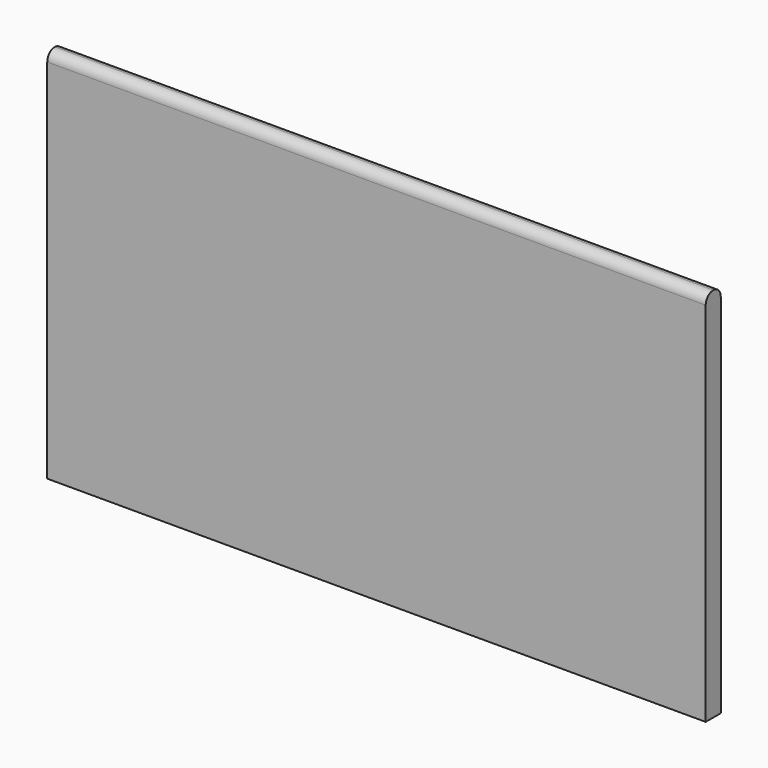
from build123d import *

# Parameters (mm, degrees)
F0_W     = 92.5
F0_H     = 20
F1_DEPTH = 1.4
F2_W     = 2
F2_H     = 2
F3_DEPTH = 25
F4_R     = 0.8
F6_W     = 70
F6_H     = 40
F7_DEPTH = 2
F8_R     = 0.99999


# Not quite as in the source:
# - a fillet or chamfer is up to 0.001 mm smaller than in the source, because OpenCascade refuses the exact size


with BuildPart() as f1:
    # F0 (on Top) → F1 (new body)
    with BuildSketch(Plane.XY):
        with Locations((46.25, 10)):
            Rectangle(F0_W, F0_H)
    extrude(amount=F1_DEPTH)

    # F2 (on face) → F3 (cut)
    with BuildSketch(Plane.XY.offset(1.4)):
        with Locations((1, 3.4)):
            Rectangle(F2_W, F2_H)
        with Locations((1, 7.8)):
            Rectangle(F2_W, F2_H)
        with Locations((1, 12.2)):
            Rectangle(F2_W, F2_H)
        with Locations((1, 16.6)):
            Rectangle(F2_W, F2_H)
    extrude(amount=-F3_DEPTH, mode=Mode.SUBTRACT)

    # F4
    f4_edges = [f1.edges().sort_by_distance(p)[0] for p in [
        (2, 15.6, 0.7),
        (2, 17.6, 0.7),
        (2, 13.2, 0.7),
        (2, 11.2, 0.7),
        (2, 6.8, 0.7),
        (2, 8.8, 0.7),
        (2, 4.4, 0.7),
        (2, 2.4, 0.7),
    ]]
    fillet(f4_edges, radius=F4_R)


with BuildPart() as f7:
    # F6 (on Front) → F7 (new body)
    with BuildSketch(Plane.XZ):
        with Locations((35, 20)):
            Rectangle(F6_W, F6_H)
    extrude(amount=F7_DEPTH)

    # F8 (radius 1 in the source; OpenCascade refuses exactly that, so slightly less here)
    f8_edges = [f7.edges().sort_by_distance(p)[0] for p in [
        (35, -2, 40),
        (35, 0, 40),
    ]]
    fillet(f8_edges, radius=F8_R)


solid = f7.part
